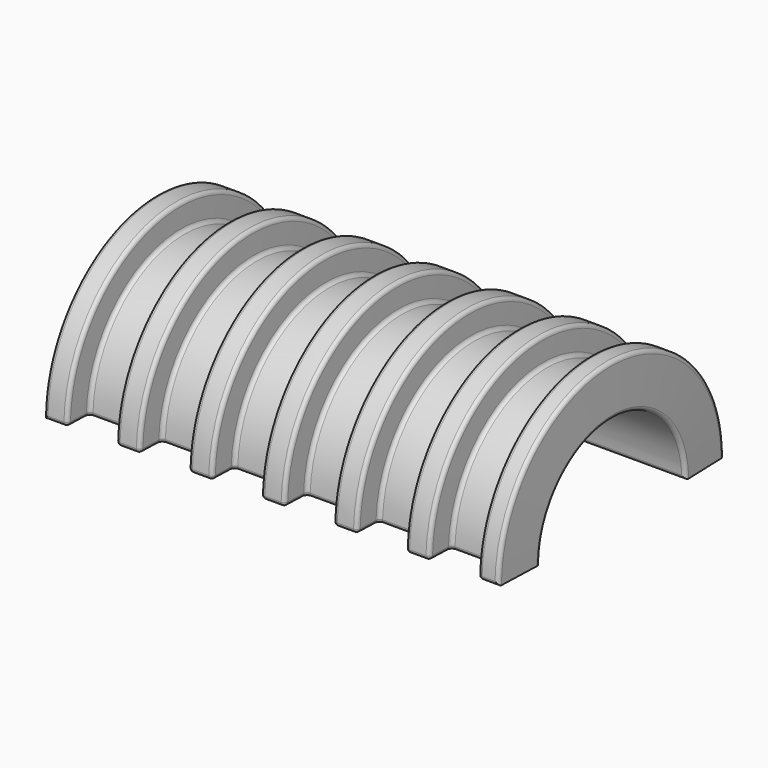
from build123d import *

# Parameters (mm, degrees)
F0_R     = 9.525
F0_R_2   = 5.5
F1_DEPTH = 31
F2_R     = 6.15
F3_DEPTH = 10.4
F4_R     = 6.65
F5_DEPTH = 9.4
F8_W     = 27.9864529148
F8_H     = 13.3397346362
F9_DEPTH = 30.9695713075
F10_R    = 0.24999


# Not quite as in the source:
# - a fillet or chamfer is up to 0.001 mm smaller than in the source, because OpenCascade refuses the exact size


with BuildPart() as f1:
    # F0 (on Right) → F1 (new body)
    with BuildSketch(Plane.YZ):
        Circle(F0_R)
        Circle(F0_R_2, mode=Mode.SUBTRACT)
    extrude(amount=-F1_DEPTH)

    # F2 (on face) → F3 (cut)
    with BuildSketch(Plane.YZ):
        Circle(F2_R)
    extrude(amount=-F3_DEPTH, mode=Mode.SUBTRACT)

    # F4 (on face) → F5 (cut)
    with BuildSketch(Plane(origin=(-31, 0, 0), x_dir=(0, -1, 0), z_dir=(-1, 0, 0))):
        Circle(F4_R)
    extrude(amount=-F5_DEPTH, mode=Mode.SUBTRACT)

    # F6 (on Front) → F7 (revolve, cut)
    with BuildSketch(Plane.XZ):
        Polygon((-1.55, 7.75), (-1.4452376915, 10.75), (-4.8452376915, 10.75), (-4.740475383, 7.75), align=None)
        Polygon((-9.640475383, 7.75), (-6.45, 7.75), (-6.3452376915, 10.75), (-9.7452376915, 10.75), align=None)
        Polygon((-14.540475383, 7.75), (-11.35, 7.75), (-11.2452376915, 10.75), (-14.6452376915, 10.75), align=None)
        Polygon((-19.440475383, 7.75), (-16.25, 7.75), (-16.1452376915, 10.75), (-19.5452376915, 10.75), align=None)
        Polygon((-24.340475383, 7.75), (-21.15, 7.75), (-21.0452376915, 10.75), (-24.4452376915, 10.75), align=None)
        Polygon((-29.240475383, 7.75), (-26.05, 7.75), (-25.9452376915, 10.75), (-29.3452376915, 10.75), align=None)
        Polygon((4.8253961525, 10.75), (-0.1746038475, 10.75), (0, 5.75), (4.8253961525, 5.75), align=None)
        Polygon((-30.8253961525, 10.75), (-35.8253961525, 10.75), (-35.8253961525, 5.75), (-31, 5.75), align=None)
    revolve(axis=Axis((-16.040995717, 0, 0), (-1, 0, 0)), mode=Mode.SUBTRACT)

    # F8 (on Right) → F9 (cut, through all)
    with BuildSketch(Plane.YZ):
        with Locations((1.1649182998, -6.6698673181)):
            Rectangle(F8_W, F8_H)
    extrude(amount=-F9_DEPTH, mode=Mode.SUBTRACT)

    # F10 (radius 0.25 in the source; OpenCascade refuses exactly that, so slightly less here)
    f10_edges = [f1.edges().sort_by_distance(p)[0] for p in [
        (-29.30246, 0, 9.525),
        (-30.085317, 9.525, 0),
        (-30.868174, 0, 9.525),
        (-30.085317, -9.525, 0),
        (-29.240475, 0, 7.75),
        (-27.645238, 7.75, 0),
        (-26.05, 0, 7.75),
        (-27.645238, -7.75, 0),
        (-24.40246, 0, 9.525),
        (-25.195238, 9.525, 0),
        (-25.988016, 0, 9.525),
        (-25.195238, -9.525, 0),
        (-24.340475, 0, 7.75),
        (-22.745238, 7.75, 0),
        (-21.15, 0, 7.75),
        (-22.745238, -7.75, 0),
        (-19.50246, 0, 9.525),
        (-20.295238, 9.525, 0),
        (-21.088016, 0, 9.525),
        (-20.295238, -9.525, 0),
        (-19.440475, 0, 7.75),
        (-17.845238, 7.75, 0),
        (-16.25, 0, 7.75),
        (-17.845238, -7.75, 0),
        (-14.60246, 0, 9.525),
        (-15.395238, 9.525, 0),
        (-16.188016, 0, 9.525),
        (-15.395238, -9.525, 0),
        (-14.540475, 0, 7.75),
        (-12.945238, 7.75, 0),
        (-11.35, 0, 7.75),
        (-12.945238, -7.75, 0),
        (-9.70246, 0, 9.525),
        (-10.495238, 9.525, 0),
        (-11.288016, 0, 9.525),
        (-10.495238, -9.525, 0),
        (-9.640475, 0, 7.75),
        (-8.045238, 7.75, 0),
        (-6.45, 0, 7.75),
        (-8.045238, -7.75, 0),
        (-4.80246, 0, 9.525),
        (-5.595238, 9.525, 0),
        (-6.388016, 0, 9.525),
        (-5.595238, -9.525, 0),
        (-4.740475, 0, 7.75),
        (-3.145238, 7.75, 0),
        (-1.55, 0, 7.75),
        (-3.145238, -7.75, 0),
        (-0.131826, 0, 9.525),
        (-0.809921, 9.525, 0),
        (-1.488016, 0, 9.525),
        (-0.809921, -9.525, 0),
        (-10.4, 0, 5.5),
        (-16, -5.5, 0),
        (-21.6, 0, 5.5),
        (-16, 5.5, 0),
        (-30.968571, 0, 6.65),
        (-26.284286, -6.65, 0),
        (-21.6, 0, 6.65),
        (-26.284286, 6.65, 0),
        (-21.6, -6.075, 0),
        (-21.6, 6.075, 0),
        (-0.013968, 0, 6.15),
        (-5.206984, 6.15, 0),
        (-10.4, 0, 6.15),
        (-5.206984, -6.15, 0),
        (-10.4, 5.825, 0),
        (-10.4, -5.825, 0),
        (-1.519008, -8.6375, 0),
        (-4.771468, -8.6375, 0),
        (-6.419008, -8.6375, 0),
        (-9.671468, -8.6375, 0),
        (-11.319008, -8.6375, 0),
        (-14.571468, -8.6375, 0),
        (-16.219008, -8.6375, 0),
        (-19.471468, -8.6375, 0),
        (-21.119008, -8.6375, 0),
        (-24.371468, -8.6375, 0),
        (-26.019008, -8.6375, 0),
        (-29.271468, -8.6375, 0),
        (-29.271468, 8.6375, 0),
        (-26.019008, 8.6375, 0),
        (-24.371468, 8.6375, 0),
        (-21.119008, 8.6375, 0),
        (-19.471468, 8.6375, 0),
        (-16.219008, 8.6375, 0),
        (-14.571468, 8.6375, 0),
        (-11.319008, 8.6375, 0),
        (-9.671468, 8.6375, 0),
        (-6.419008, 8.6375, 0),
        (-4.771468, 8.6375, 0),
        (-1.519008, 8.6375, 0),
    ]]
    fillet(f10_edges, radius=F10_R)


solid = f1.part
